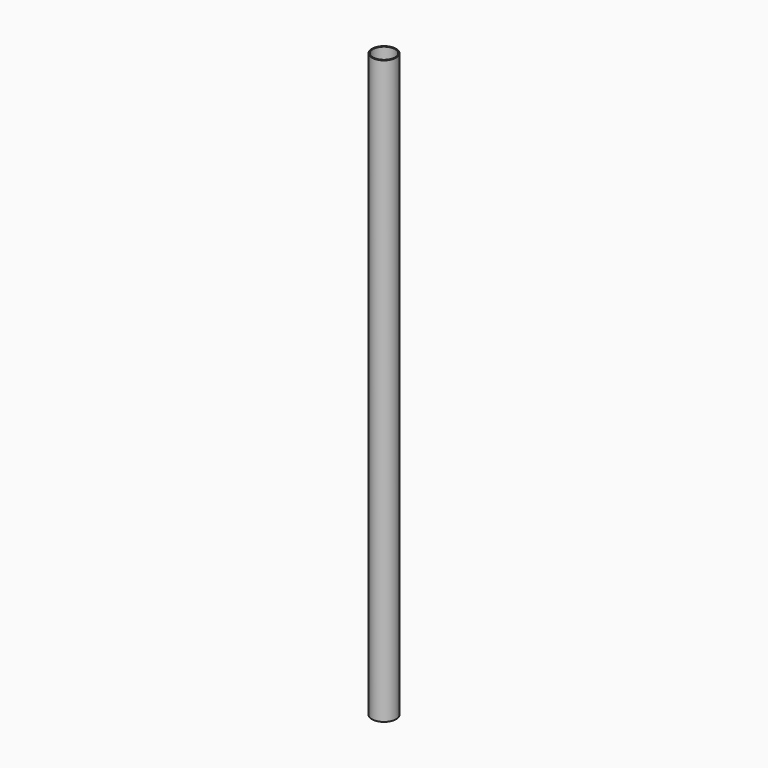
from build123d import *

# Parameters (mm, degrees)
F0_R     = 19.05
F1_DEPTH = 914.4
F3_D     = 34.798


# Not quite as in the source:
# - the program builds the solid bodies; features that only make, move or delete a surface that nothing else refers to are left out


with BuildPart() as f1:
    # F0 (on Top) → F1 (new body)
    with BuildSketch(Plane.XY):
        Circle(F0_R)
    extrude(amount=F1_DEPTH)

    # F3 (through all)
    with Locations(Plane.XY.offset(914.4)):
        with Locations((0, 0)):
            Hole(F3_D / 2)


solid = f1.part
